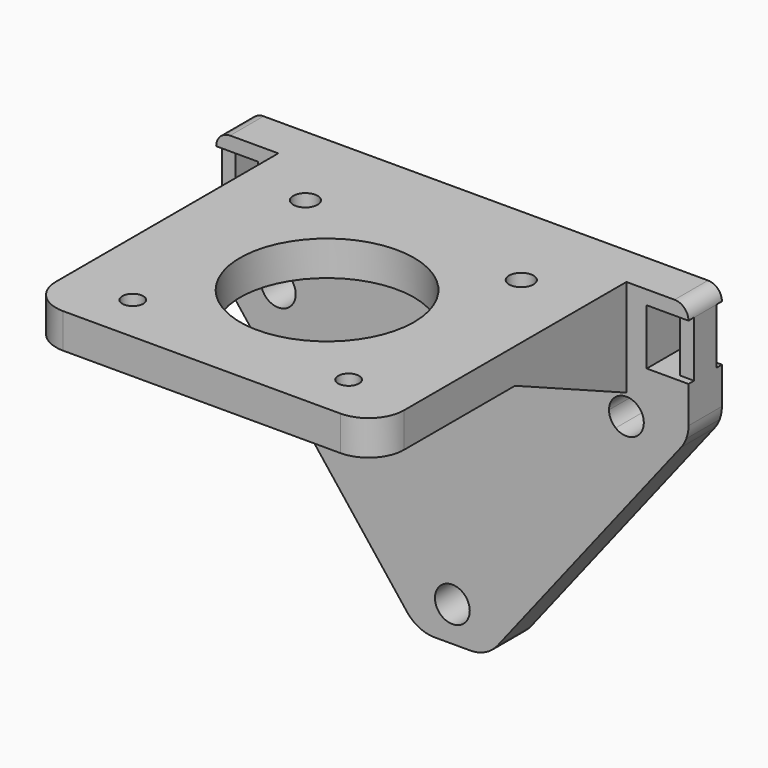
from build123d import *

# Parameters (mm, degrees)
F0_W      = 4
F0_H      = 8
F0_W_2    = 2
F1_DEPTH  = 6
F2_W      = 2
F2_H      = 8
F3_DEPTH  = 1
F4_W      = 2
F4_H      = 8
F5_DEPTH  = 1
F6_W      = 25
F6_H      = 5
F7_DEPTH  = 45
F8_R      = 5.08
F9_W      = 2.5
F9_H      = 20
F10_DEPTH = 9
F12_DEPTH = 50.292
F13_R     = 12.5
F13_R_2   = 1.75
F13_R_3   = 1.5
F14_DEPTH = 25.4


# Not quite as in the source:
# - a feature names something its author has since deleted; it is built from what else it names


with BuildPart() as f1:
    # F0 (on Front) → F1 (new body)
    with BuildSketch(Plane.XZ):
        with BuildLine():
            Line((-22.5, 15.1779663801), (-15.95, 15.1779663801))
            Line((-15.95, 15.1779663801), (15.95, 15.1779663801))
            Line((15.95, 15.1779663801), (22.5, 15.1779663801))
            ThreePointArc((22.5, 15.1779663801), (25, 17.6779663801), (27.5, 15.1779663801))
            Line((27.5, 15.1779663801), (33.6112053721, 15.1779663801))
            ThreePointArc((33.6112053721, 15.1779663801), (33.8410734014, 16.027307097), (33.9184952978, 16.9037914461))
            Line((33.9184952978, 16.9037914461), (33.9184952978, 19.2973875134))
            Line((33.9184952978, 19.2973875134), (33.9184952978, 20.1779663801))
            Line((33.9184952978, 20.1779663801), (33.0379164311, 20.1779663801))
            Line((33.0379164311, 20.1779663801), (-32.6408470514, 20.1779663801))
            Line((-32.6408470514, 20.1779663801), (-33.9184952978, 20.1779663801))
            Line((-33.9184952978, 20.1779663801), (-33.9184952978, 18.9003181337))
            Line((-33.9184952978, 18.9003181337), (-33.9184952978, 16.9037914461))
            ThreePointArc((-33.9184952978, 16.9037914461), (-33.8410734014, 16.027307097), (-33.6112053721, 15.1779663801))
            Line((-33.6112053721, 15.1779663801), (-27.5, 15.1779663801))
            ThreePointArc((-27.5, 15.1779663801), (-25, 17.6779663801), (-22.5, 15.1779663801))
        make_face()
        with BuildLine():
            Line((15.95, 15.1779663801), (-15.95, 15.1779663801))
            Line((-15.95, 15.1779663801), (-22.5, 15.1779663801))
            ThreePointArc((-22.5, 15.1779663801), (-22.7521952698, 14.0837205691), (-23.457899116, 13.2102456521))
            Line((-23.457899116, 13.2102456521), (-1.542100884, -14.7543128919))
            ThreePointArc((-1.542100884, -14.7543128919), (0, -14.2220336199), (1.542100884, -14.7543128919))
            Line((1.542100884, -14.7543128919), (23.457899116, 13.2102456521))
            ThreePointArc((23.457899116, 13.2102456521), (22.7521952698, 14.0837205691), (22.5, 15.1779663801))
            Line((22.5, 15.1779663801), (15.95, 15.1779663801))
        make_face()
        with BuildLine():
            ThreePointArc((-23.457899116, 13.2102456521), (-26.094245811, 12.9301616499), (-27.5, 15.1779663801))
            Line((-27.5, 15.1779663801), (-33.6112053721, 15.1779663801))
            ThreePointArc((-33.6112053721, 15.1779663801), (-33.28570797, 14.4691552359), (-32.8539367538, 13.819589678))
            Line((-32.8539367538, 13.819589678), (-6.5014092727, -19.8062353879))
            ThreePointArc((-6.5014092727, -19.8062353879), (-4.7544594387, -21.2176430802), (-2.5659678166, -21.7220336199))
            Line((-2.5659678166, -21.7220336199), (0, -21.7220336199))
            Line((0, -21.7220336199), (0, -19.2220336199))
            ThreePointArc((0, -19.2220336199), (-2.3631866008, -17.5377229541), (-1.542100884, -14.7543128919))
            Line((-1.542100884, -14.7543128919), (-23.457899116, 13.2102456521))
        make_face()
        with BuildLine():
            Line((33.6112053721, 15.1779663801), (27.5, 15.1779663801))
            ThreePointArc((27.5, 15.1779663801), (26.094245811, 12.9301616499), (23.457899116, 13.2102456521))
            Line((23.457899116, 13.2102456521), (1.542100884, -14.7543128919))
            ThreePointArc((1.542100884, -14.7543128919), (2.2478047302, -15.6277878088), (2.5, -16.7220336199))
            ThreePointArc((2.5, -16.7220336199), (1.767766953, -18.4898005728), (0, -19.2220336199))
            Line((0, -19.2220336199), (0, -21.7220336199))
            Line((0, -21.7220336199), (2.5659678166, -21.7220336199))
            ThreePointArc((2.5659678166, -21.7220336199), (4.7544594387, -21.2176430802), (6.5014092727, -19.8062353879))
            Line((6.5014092727, -19.8062353879), (32.8539367538, 13.819589678))
            ThreePointArc((32.8539367538, 13.819589678), (33.28570797, 14.4691552359), (33.6112053721, 15.1779663801))
        make_face()
        with BuildLine():
            Line((-33.9184952978, 30.1779663801), (-33.9184952978, 20.1779663801))
            Line((-33.9184952978, 20.1779663801), (-32.6408470514, 20.1779663801))
            Line((-32.6408470514, 20.1779663801), (33.0379164311, 20.1779663801))
            Line((33.0379164311, 20.1779663801), (33.9184952978, 20.1779663801))
            Line((33.9184952978, 20.1779663801), (33.9184952978, 22.1779663801))
            Line((33.9184952978, 22.1779663801), (31.9184952978, 22.1779663801))
            Line((31.9184952978, 22.1779663801), (27.9184952978, 22.1779663801))
            Line((27.9184952978, 22.1779663801), (27.9184952978, 30.1779663801))
            Line((27.9184952978, 30.1779663801), (31.9184952978, 30.1779663801))
            Line((31.9184952978, 30.1779663801), (33.9184952978, 30.1779663801))
            ThreePointArc((33.9184952978, 30.1779663801), (33.3327088602, 31.5921799425), (31.9184952978, 32.1779663801))
            Line((31.9184952978, 32.1779663801), (-31.9184952978, 32.1779663801))
            ThreePointArc((-31.9184952978, 32.1779663801), (-33.3327088602, 31.5921799425), (-33.9184952978, 30.1779663801))
        make_face()
        with Locations((-29.9184952978, 26.1779663801)):
            Rectangle(F0_W, F0_H, mode=Mode.SUBTRACT)
        with Locations((32.9184952978, 26.1779663801)):
            Rectangle(F0_W_2, F0_H)
    extrude(amount=F1_DEPTH)

    # F2 (on face) → F3 (cut)
    with BuildSketch(Plane(origin=(0, 0, 0), x_dir=(-1, 0, 0), z_dir=(0, 1, 0))):
        with Locations((-32.9184952978, 26.1779663801)):
            Rectangle(F2_W, F2_H)
        with Locations((32.9184952978, 26.1779663801)):
            Rectangle(F2_W, F2_H)
    extrude(amount=-F3_DEPTH, mode=Mode.SUBTRACT)

    # F4 (on face) → F5 (cut)
    with BuildSketch(Plane.XZ.offset(6)):
        with Locations((-32.9184952978, 26.1779663801)):
            Rectangle(F4_W, F4_H)
        with Locations((32.9184952978, 26.1779663801)):
            Rectangle(F4_W, F4_H)
    extrude(amount=-F5_DEPTH, mode=Mode.SUBTRACT)

    # F6 (on face) → F7 (join)
    with BuildSketch(Plane.XZ.offset(6)):
        with Locations((-12.5, 29.6779663801)):
            Rectangle(F6_W, F6_H)
        with Locations((12.5, 29.6779663801)):
            Rectangle(F6_W, F6_H)
    extrude(amount=F7_DEPTH)

    # F8
    f8_edges = [f1.edges().sort_by_distance(p)[0] for p in [
        (25, -51, 29.677966),
        (-25, -51, 29.677966),
    ]]
    fillet(f8_edges, radius=F8_R)

    # F9 (on face) → F10 (join)
    with BuildSketch(Plane(origin=(0, 0, 27.1779663801), x_dir=(1, 0, 0), z_dir=(0, 0, -1))):
        with Locations((23.75, 16)):
            Rectangle(F9_W, F9_H)
        with Locations((-23.75, 16)):
            Rectangle(F9_W, F9_H)
    extrude(amount=F10_DEPTH)

    # F11 (on face) → F12 (cut)
    with BuildSketch(Plane(origin=(-25, 0, 0), x_dir=(0, -1, 0), z_dir=(-1, 0, 0))):
        Polygon((26, 27.1779663801), (6, 18.1779663801), (26, 18.1779663801), align=None)
    extrude(amount=-F12_DEPTH, mode=Mode.SUBTRACT)

    # F13 (on face) → F14 (cut)
    with BuildSketch(Plane.XY.offset(32.1779663801)):
        with Locations((0, -28.5)):
            Circle(F13_R)
        with Locations((-15.5, -13)):
            Circle(F13_R_2)
        with Locations((15.5, -13)):
            Circle(F13_R_2)
        with Locations((15.5, -44)):
            Circle(F13_R_3)
        with Locations((-15.5, -44)):
            Circle(F13_R_3)
    extrude(amount=-F14_DEPTH, mode=Mode.SUBTRACT)


solid = f1.part
